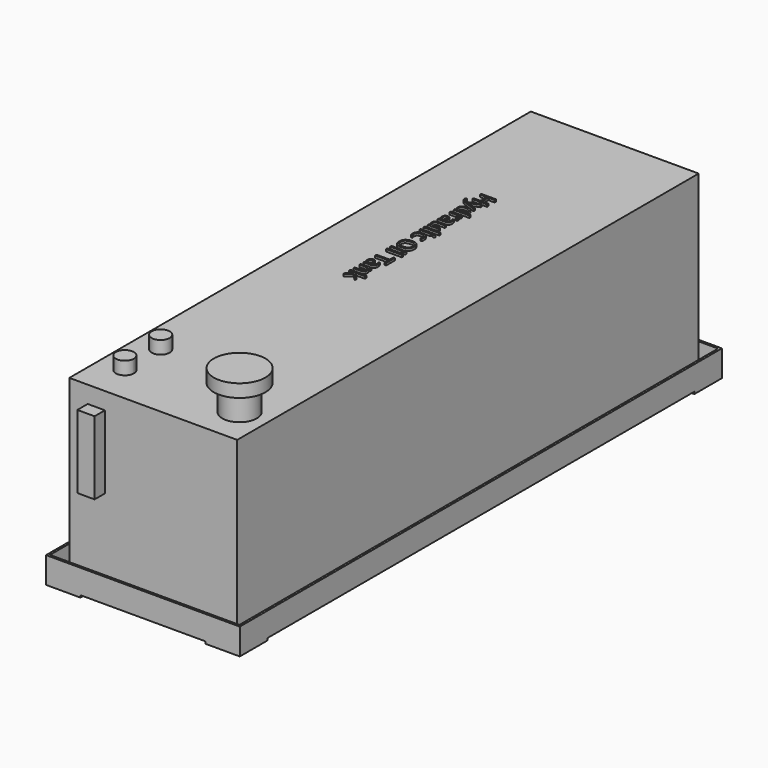
from build123d import *

# Parameters (mm, degrees)
F0_W         = 390
F0_H         = 410
F1_DEPTH     = 1340
F2_W         = 450
F2_H         = 1400
F2_W_2       = 390
F2_H_2       = 1340
F3_DEPTH     = 6
F4_W         = 450
F4_H         = 1400
F4_W_2       = 440
F4_H_2       = 1390
F5_DEPTH     = 50
F6_W         = 40
F6_H         = 170
F7_DEPTH     = 30
F8_R         = 40
F9_DEPTH     = 60
F10_DEPTH    = 30
F8_TEXT_SIZE = 48.0386487165
F11_DEPTH    = 5
F12_R        = 60
F12_R_2      = 40
F13_DEPTH    = 30
F14_W        = 80
F14_H        = 80
F15_DEPTH    = 5


# Not quite as in the source:
# - Text() gives the source's letters only with a copy of the font that has no kerning and outlines rounded to 1/6400 em; it was checked with that copy


with BuildPart() as f1:
    # F0 (on Front) → F1 (new body)
    with BuildSketch(Plane.XZ):
        with Locations((195, 205)):
            Rectangle(F0_W, F0_H)
    extrude(amount=-F1_DEPTH)

    # F2 (on face) → F3 (join)
    with BuildSketch(Plane(origin=(0, 0, 0), x_dir=(1, 0, 0), z_dir=(0, 0, -1))):
        with Locations((195, -670)):
            Rectangle(F2_W, F2_H)
        with Locations((195, -670)):
            Rectangle(F2_W_2, F2_H_2, mode=Mode.SUBTRACT)
        with Locations((195, -670)):
            Rectangle(F2_W_2, F2_H_2)
    extrude(amount=F3_DEPTH)

    # F4 (on face) → F5 (join)
    with BuildSketch(Plane.XY):
        with Locations((195, 670)):
            Rectangle(F4_W, F4_H)
        with Locations((195, 670)):
            Rectangle(F4_W_2, F4_H_2, mode=Mode.SUBTRACT)
    extrude(amount=F5_DEPTH)

    # F6 (on face) → F7 (join)
    with BuildSketch(Plane.XZ):
        with Locations((62.6989039779, 285.5376815796)):
            Rectangle(F6_W, F6_H)
    extrude(amount=F7_DEPTH)

    # F8 (on face) → F9 (join)
    with BuildSketch(Plane.XY.offset(410)):
        with Locations((325.0986337662, 88.0740657449)):
            Circle(F8_R)
    extrude(amount=F9_DEPTH)

    # F8 (on face) → F10 (join)
    with BuildSketch(Plane.XY.offset(410)):
        with BuildLine():
            ThreePointArc((80.4247952104, 191.0568028688), (44.5755528054, 205.9060452738), (59.4247952104, 170.0568028688))
            ThreePointArc((59.4247952104, 170.0568028688), (74.2740376153, 176.2075604639), (80.4247952104, 191.0568028688))
        make_face()
        with BuildLine():
            ThreePointArc((59.4247952104, 107.9365930557), (44.5755528054, 72.0873506508), (80.4247952104, 86.9365930557))
            ThreePointArc((80.4247952104, 86.9365930557), (74.2740376153, 101.7858354606), (59.4247952104, 107.9365930557))
        make_face()
    extrude(amount=F10_DEPTH)

    # F8 (on face) → F11 (join)
    with BuildSketch(Plane.XY.offset(410)):
        with BuildLine():
            ThreePointArc((59.4247952104, 107.9365930557), (44.5755528054, 72.0873506508), (80.4247952104, 86.9365930557))
            ThreePointArc((80.4247952104, 86.9365930557), (74.2740376153, 101.7858354606), (59.4247952104, 107.9365930557))
        make_face()
        with BuildLine():
            ThreePointArc((80.4247952104, 191.0568028688), (44.5755528054, 205.9060452738), (59.4247952104, 170.0568028688))
            ThreePointArc((59.4247952104, 170.0568028688), (74.2740376153, 176.2075604639), (80.4247952104, 191.0568028688))
        make_face()
        with Locations((325.0986337662, 88.0740657449)):
            Circle(F8_R)
        with Locations(Location((137.7631242778, 1028.4524796512), (0, 0, -89.8216209195))):
            Text('Hydraulic Oil Tank', F8_TEXT_SIZE, font='Open Sans', text_align=(TextAlign.LEFT, TextAlign.BOTTOM))
    extrude(amount=F11_DEPTH)

    # F12 (on face) → F13 (join)
    with BuildSketch(Plane.XY.offset(470)):
        with Locations((325.0986337662, 88.0740657449)):
            Circle(F12_R)
        with Locations((325.0986337662, 88.0740657449)):
            Circle(F12_R_2, mode=Mode.SUBTRACT)
        with Locations((325.0986337662, 88.0740657449)):
            Circle(F12_R_2)
    extrude(amount=F13_DEPTH)

    # F14 (on face) → F15 (join)
    with BuildSketch(Plane(origin=(0, 0, -6), x_dir=(1, 0, 0), z_dir=(0, 0, -1))):
        with Locations((380, -10)):
            Rectangle(F14_W, F14_H)
        with Locations((380, -1330)):
            Rectangle(F14_W, F14_H)
        with Locations((10, -1330)):
            Rectangle(F14_W, F14_H)
        with Locations((10, -10)):
            Rectangle(F14_W, F14_H)
    extrude(amount=F15_DEPTH)


solid = f1.part
